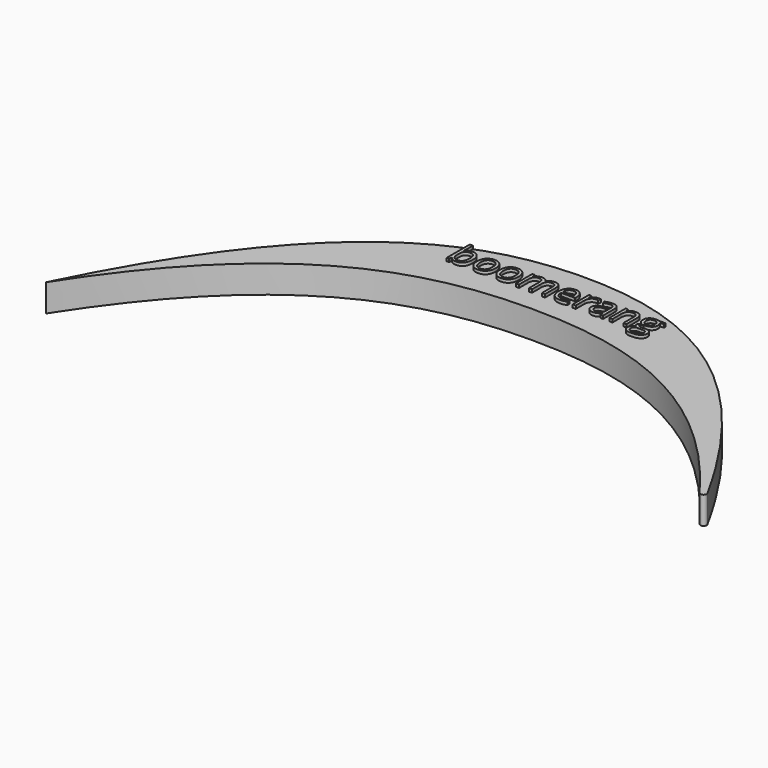
from build123d import *

# Parameters (mm, degrees)
F1_DEPTH     = 9
F2_TEXT_SIZE = 12.4347590506
F3_DEPTH     = 1


# Not quite as in the source:
# - Text() gives the source's letters only with a copy of the font that has no kerning and outlines rounded to 1/6400 em; it was checked with that copy


with BuildPart() as f1:
    # F0 (on Top) → F1 (new body)
    with BuildSketch(Plane.XY):
        with BuildLine():
            Line((59.2199351302, 33), (0, 33))
            add(Edge.make_bspline(
                [(0, 33), (32.3126732762, 33.0000022693), (64.6253465523, 23.8376536016), (96.9380198285, -19.7238664553)],
                knots=[0.5, 0.5, 0.5, 0.5, 0.9568750789, 0.9568750789, 0.9568750789, 0.9568750789], degree=3))
            ThreePointArc((96.9380198285, -19.7238664553), (98.281635619, -19.9694779321), (98.6169640405, -18.6453996716))
            add(Edge.make_bspline(
                [(59.2199351302, 33), (72.3522781003, 21.7237770143), (85.4846210704, 5.1809148278), (98.6169640405, -18.6453996716)],
                knots=[0.7791073367, 0.7791073367, 0.7791073367, 0.7791073367, 0.9647880503, 0.9647880503, 0.9647880503, 0.9647880503], degree=3))
        make_face()
        with BuildLine():
            add(Edge.make_bspline(
                [(-106.0881018639, -33), (-90.4653818422, -1.2827657722), (-74.8426618205, 19.5853868586), (-59.2199417988, 33)],
                knots=[0, 0, 0, 0, 0.2208926319, 0.2208926319, 0.2208926319, 0.2208926319], degree=3))
            add(Edge.make_bspline(
                [(-106.0881018639, -33), (-70.7254012426, 22.0263226032), (-35.3627006213, 32.9999975165), (0, 33)],
                knots=[0, 0, 0, 0, 0.5, 0.5, 0.5, 0.5], degree=3))
            Line((0, 33), (-59.2199417988, 33))
        make_face()
        with BuildLine():
            Line((0, 55), (0, 33))
            Line((0, 33), (59.2199351302, 33))
            add(Edge.make_bspline(
                [(0, 55), (19.7399783767, 54.9999986137), (39.4799567534, 49.9499379064), (59.2199351302, 33)],
                knots=[0.5, 0.5, 0.5, 0.5, 0.7791073367, 0.7791073367, 0.7791073367, 0.7791073367], degree=3))
        make_face()
        with BuildLine():
            Line((-59.2199417988, 33), (0, 33))
            Line((0, 33), (0, 55))
            add(Edge.make_bspline(
                [(-59.2199417988, 33), (-39.4799611992, 49.9499423144), (-19.7399805996, 55.0000013863), (0, 55)],
                knots=[0.2208926319, 0.2208926319, 0.2208926319, 0.2208926319, 0.5, 0.5, 0.5, 0.5], degree=3))
        make_face()
    extrude(amount=F1_DEPTH)


with BuildPart() as f3:
    # F2 (on face) → F3 (new body)
    with BuildSketch(Plane.XY.offset(9)):
        with Locations((-34.5394350915, 39.9222438286)):
            Text('boomerang', F2_TEXT_SIZE, font='Open Sans', text_align=(TextAlign.LEFT, TextAlign.BOTTOM))
    extrude(amount=F3_DEPTH)


solid = Compound([f1.part, f3.part])
